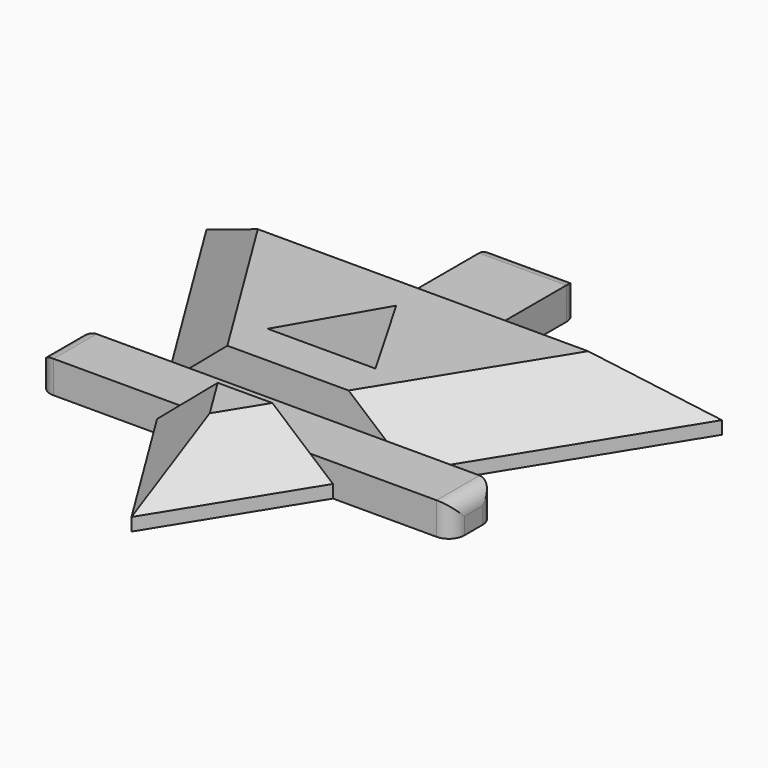
from build123d import *

# Parameters (mm, degrees)
F1_DEPTH     = 3.175
F2_W         = 20.397445187
F2_H         = 2.647349927
F2_W_2       = 4.2995549738
F2_H_2       = 13.8314400401
F3_DEPTH     = 1.5875
F4_W         = 14.3783436368
F4_H         = 2.647349927
F5_DEPTH     = 25.4
F6_T4_DEPTH  = 25.8319450188
F6_T9_DEPTH  = 25.8319450188
F6_T14_DEPTH = 38.4641495789
F6_T19_DEPTH = 38.4641495789
F6_T24_DEPTH = 38.4641495789
F6_T29_DEPTH = 25.8319450188
F6_T34_DEPTH = 25.8319450188
F6_T39_DEPTH = 21.2914590052
F6_T44_DEPTH = 21.2914590052
F6_T49_DEPTH = 21.2914590052
F6_T54_DEPTH = 21.2914590052
F7_R         = 0.762
F9_DEPTH     = 25.4


# Not quite as in the source:
# - a fillet or chamfer that OpenCascade refuses, or shapes differently, is made with other operations: its cross-section is extruded or revolved along the edge and cut away or added


with BuildPart() as f1:
    # F0 (on Top) → F1 (new body)
    with BuildSketch(Plane.XY):
        Polygon((12.7, 7.7934656292), (-12.7, 7.7934656292), (0, -12.7), align=None)
    extrude(amount=F1_DEPTH)

    # F2 (on Top) → F3 (join)
    with BuildSketch(Plane.XY):
        with Locations((0, -4.3830036468)):
            Rectangle(F2_W, F2_H)
        with Locations((0, 5.2467339706)):
            Rectangle(F2_W_2, F2_H_2)
    extrude(amount=F3_DEPTH)

    # F4 (on face) → F5 (cut)
    with BuildSketch(Plane.XY.offset(1.5875)):
        with Locations((-1.2147540241, -4.3830036468)):
            Rectangle(F4_W, F4_H)
    extrude(amount=F5_DEPTH, mode=Mode.SUBTRACT)

    # F6: chamfer of 2.54 on 5 edges, made by hand


with BuildPart() as f6_tool2:
    # F6_s3 → F6_t4 (new body)
    with BuildSketch(Plane(origin=(-10.454367288, 16.8697808418, 0), x_dir=(0, 0, 1), z_dir=(0.5267614317, -0.8500131729, 0))):
        Polygon((0.635, 6.6898701827), (3.175, 4.1498701827), (3.175, 6.6898701827), align=None)
    extrude(amount=F6_T4_DEPTH)

    split(bisect_by=Plane.XZ.offset(3.0593286833), keep=Keep.BOTTOM)


with BuildPart() as f1_1:
    add(f1.part)

    # F6_t1: cut F6_tool2
    add(f6_tool2.part, mode=Mode.SUBTRACT)


with BuildPart() as f6_tool7:
    # F6_s8 → F6_t9 (new body)
    with BuildSketch(Plane(origin=(-10.454367288, 16.8697808418, 0), x_dir=(0, 0, 1), z_dir=(0.5267614317, -0.8500131729, 0))):
        Polygon((0.635, 6.6898701827), (3.175, 4.1498701827), (3.175, 6.6898701827), align=None)
    extrude(amount=F6_T9_DEPTH)

    split(bisect_by=Plane.XZ.offset(5.7066786103), keep=Keep.TOP)


with BuildPart() as f1_2:
    add(f1_1.part)

    # F6_t6: cut F6_tool7
    add(f6_tool7.part, mode=Mode.SUBTRACT)


with BuildPart() as f6_tool12:
    # F6_s13 → F6_t14 (new body)
    with BuildSketch(Plane.YZ.offset(19.2320747894)):
        Polygon((7.7934656292, 0.635), (5.2534656292, 3.175), (7.7934656292, 3.175), align=None)
    extrude(amount=-F6_T14_DEPTH)

    split(bisect_by=Plane.YZ.offset(2.1497774869), keep=Keep.TOP)


with BuildPart() as f1_3:
    add(f1_2.part)

    # F6_t11: cut F6_tool12
    add(f6_tool12.part, mode=Mode.SUBTRACT)


with BuildPart() as f6_tool17:
    # F6_s18 → F6_t19 (new body)
    with BuildSketch(Plane.YZ.offset(19.2320747894)):
        Polygon((7.7934656292, 0.635), (5.2534656292, 3.175), (7.7934656292, 3.175), align=None)
    extrude(amount=-F6_T19_DEPTH)

    split(bisect_by=Plane.XY.offset(1.5875), keep=Keep.TOP)


with BuildPart() as f1_4:
    add(f1_3.part)

    # F6_t16: cut F6_tool17
    add(f6_tool17.part, mode=Mode.SUBTRACT)


with BuildPart() as f6_tool22:
    # F6_s23 → F6_t24 (new body)
    with BuildSketch(Plane.YZ.offset(19.2320747894)):
        Polygon((7.7934656292, 0.635), (5.2534656292, 3.175), (7.7934656292, 3.175), align=None)
    extrude(amount=-F6_T24_DEPTH)

    split(bisect_by=Plane.YZ.offset(-2.1497774869), keep=Keep.BOTTOM)


with BuildPart() as f1_5:
    add(f1_4.part)

    # F6_t21: cut F6_tool22
    add(f6_tool22.part, mode=Mode.SUBTRACT)


with BuildPart() as f6_tool27:
    # F6_s28 → F6_t29 (new body)
    with BuildSketch(Plane(origin=(-3.1529050539, -5.0877127051, 0), x_dir=(0, 0, 1), z_dir=(0.5267614317, 0.8500131729, 0))):
        Polygon((0.635, 6.6898701827), (3.175, 4.1498701827), (3.175, 6.6898701827), align=None)
    extrude(amount=F6_T29_DEPTH)

    split(bisect_by=Plane.XZ.offset(5.7066786103), keep=Keep.TOP)


with BuildPart() as f1_6:
    add(f1_5.part)

    # F6_t26: cut F6_tool27
    add(f6_tool27.part, mode=Mode.SUBTRACT)


with BuildPart() as f6_tool32:
    # F6_s33 → F6_t34 (new body)
    with BuildSketch(Plane(origin=(-3.1529050539, -5.0877127051, 0), x_dir=(0, 0, 1), z_dir=(0.5267614317, 0.8500131729, 0))):
        Polygon((0.635, 6.6898701827), (3.175, 4.1498701827), (3.175, 6.6898701827), align=None)
    extrude(amount=F6_T34_DEPTH)

    split(bisect_by=Plane.XZ.offset(3.0593286833), keep=Keep.BOTTOM)


with BuildPart() as f1_7:
    add(f1_6.part)

    # F6_t31: cut F6_tool32
    add(f6_tool32.part, mode=Mode.SUBTRACT)


with BuildPart() as f6_tool37:
    # F6_s38 → F6_t39 (new body)
    with BuildSketch(Plane(origin=(-9.1273228482, -14.7283840218, 0), x_dir=(0, 0, 1), z_dir=(0.5267614317, 0.8500131729, 0))):
        Polygon((0.635, 6.6898701827), (3.175, 4.1498701827), (3.175, 6.6898701827), align=None)
    extrude(amount=F6_T39_DEPTH)

    split(bisect_by=Plane.XZ.offset(5.7066786103), keep=Keep.TOP)


with BuildPart() as f1_8:
    add(f1_7.part)

    # F6_t36: cut F6_tool37
    add(f6_tool37.part, mode=Mode.SUBTRACT)


with BuildPart() as f6_tool42:
    # F6_s43 → F6_t44 (new body)
    with BuildSketch(Plane(origin=(-9.1273228482, -14.7283840218, 0), x_dir=(0, 0, 1), z_dir=(0.5267614317, 0.8500131729, 0))):
        Polygon((0.635, 6.6898701827), (3.175, 4.1498701827), (3.175, 6.6898701827), align=None)
    extrude(amount=F6_T44_DEPTH)

    split(bisect_by=Plane.XZ.offset(3.0593286833), keep=Keep.BOTTOM)


with BuildPart() as f1_9:
    add(f1_8.part)

    # F6_t41: cut F6_tool42
    add(f6_tool42.part, mode=Mode.SUBTRACT)


with BuildPart() as f6_tool47:
    # F6_s48 → F6_t49 (new body)
    with BuildSketch(Plane(origin=(-2.0881965805, 3.3696366023, 0), x_dir=(0, 0, 1), z_dir=(0.5267614317, -0.8500131729, 0))):
        Polygon((0.635, 6.6898701827), (3.175, 4.1498701827), (3.175, 6.6898701827), align=None)
    extrude(amount=F6_T49_DEPTH)

    split(bisect_by=Plane.XZ.offset(3.0593286833), keep=Keep.BOTTOM)


with BuildPart() as f1_10:
    add(f1_9.part)

    # F6_t46: cut F6_tool47
    add(f6_tool47.part, mode=Mode.SUBTRACT)


with BuildPart() as f6_tool52:
    # F6_s53 → F6_t54 (new body)
    with BuildSketch(Plane(origin=(-2.0881965805, 3.3696366023, 0), x_dir=(0, 0, 1), z_dir=(0.5267614317, -0.8500131729, 0))):
        Polygon((0.635, 6.6898701827), (3.175, 4.1498701827), (3.175, 6.6898701827), align=None)
    extrude(amount=F6_T54_DEPTH)

    split(bisect_by=Plane.XZ.offset(5.7066786103), keep=Keep.TOP)


with BuildPart() as f1_11:
    add(f1_10.part)

    # F6_t51: cut F6_tool52
    add(f6_tool52.part, mode=Mode.SUBTRACT)

    # F7
    f7_edges = [f1_11.edges().sort_by_distance(p)[0] for p in [
        (-2.149777, 12.162454, 0.79375),
        (0, 12.162454, 1.5875),
        (2.149777, 12.162454, 0.79375),
        (-10.198723, -4.383004, 1.5875),
        (-10.198723, -5.706679, 0.79375),
        (-10.198723, -3.059329, 0.79375),
        (10.198723, -3.059329, 0.79375),
        (10.198723, -5.706679, 0.79375),
        (10.198723, -4.383004, 1.5875),
    ]]
    fillet(f7_edges, radius=F7_R)

    # F8 (on face) → F9 (cut)
    with BuildSketch(Plane.XY.offset(3.175)):
        Polygon((-2.6549665111, -0.989894278), (0, -0.989894278), (2.6549665111, -0.989894278), (0, 3.6086426117), align=None)
    extrude(amount=-F9_DEPTH, mode=Mode.SUBTRACT)


solid = f1_11.part
